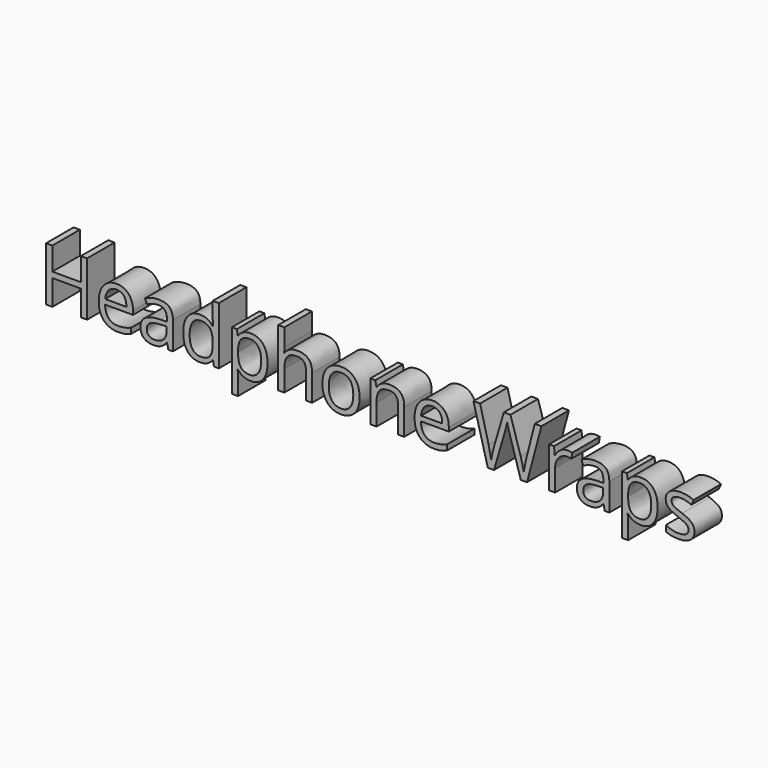
from build123d import *

# Parameters (mm, degrees)
F0_TEXT_SIZE = 55.9101993632
F1_DEPTH     = 25.4


# Not quite as in the source:
# - Text() gives the source's letters only with a copy of the font that has no kerning and outlines rounded to 1/6400 em; it was checked with that copy


with BuildPart() as f1:
    # F0 (on Front) → F1 (new body)
    with BuildSketch(Plane.XZ):
        with Locations((-175.2586886287, -12.5750591978)):
            Text('Headphone Wraps', F0_TEXT_SIZE, font='Open Sans', text_align=(TextAlign.LEFT, TextAlign.BOTTOM))
    extrude(amount=F1_DEPTH)


solid = f1.part
